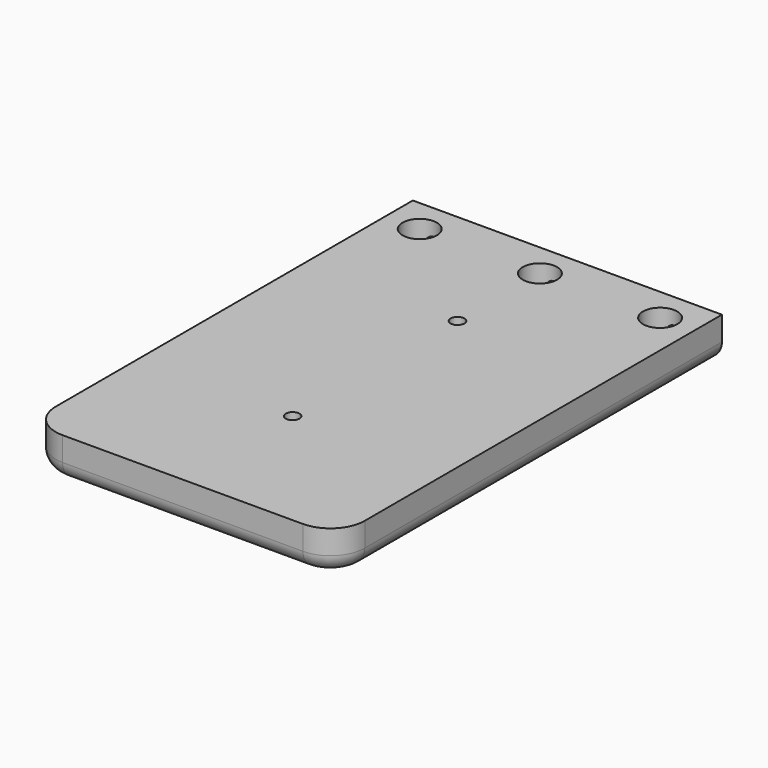
from build123d import *

# Parameters (mm, degrees)
F0_R     = 2
F0_R_2   = 5
F1_DEPTH = 12
F2_R     = 2
F3_DEPTH = 25
F4_R     = 4.99999


# Not quite as in the source:
# - a fillet or chamfer is up to 0.001 mm smaller than in the source, because OpenCascade refuses the exact size


with BuildPart() as f1:
    # F0 (on Top) → F1 (new body)
    with BuildSketch(Plane.XY):
        with BuildLine():
            Line((-35.0000017881, -70), (35.0000017881, -70))
            ThreePointArc((35.0000017881, -70), (42.0710696, -67.0710678119), (45.0000017881, -60))
            Line((45.0000017881, -60), (45.0000017881, 70))
            Line((45.0000017881, 70), (-45.0000017881, 70))
            Line((-45.0000017881, 70), (-45.0000017881, -60))
            ThreePointArc((-45.0000017881, -60), (-42.0710696, -67.0710678119), (-35.0000017881, -70))
        make_face()
        with Locations((0, -30)):
            Circle(F0_R, mode=Mode.SUBTRACT)
        with Locations((0, 30)):
            Circle(F0_R, mode=Mode.SUBTRACT)
        with Locations((-35.0000017881, 60)):
            Circle(F0_R_2, mode=Mode.SUBTRACT)
        with Locations((0, 60)):
            Circle(F0_R_2, mode=Mode.SUBTRACT)
        with Locations((35.0000017881, 60)):
            Circle(F0_R_2, mode=Mode.SUBTRACT)
    extrude(amount=F1_DEPTH)

    # F2 (on face) → F3 (cut)
    with BuildSketch(Plane(origin=(0, 70, 0), x_dir=(-1, 0, 0), z_dir=(0, 1, 0))):
        with Locations((0, 6)):
            Circle(F2_R)
        with Locations((35.0000017881, 6)):
            Circle(F2_R)
        with Locations((-35.0000017881, 6)):
            Circle(F2_R)
    extrude(amount=-F3_DEPTH, mode=Mode.SUBTRACT)

    # F4 (radius 5 in the source; OpenCascade refuses exactly that, so slightly less here)
    f4_edges = [f1.edges().sort_by_distance(p)[0] for p in [
        (45.000002, 5, 0),
    ]]
    fillet(f4_edges, radius=F4_R)


solid = f1.part
